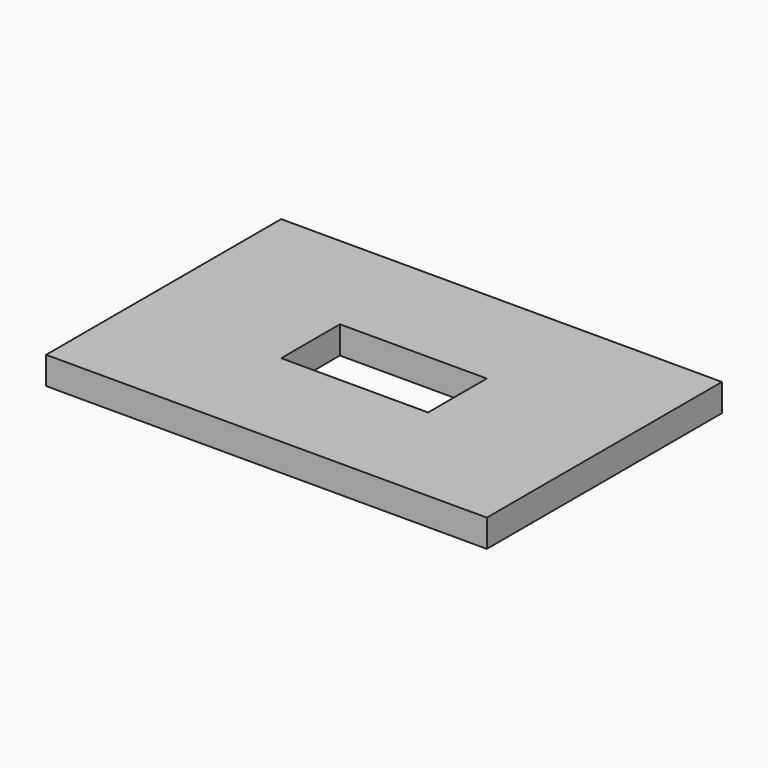
from build123d import *

# Parameters (mm, degrees)
F0_W     = 152.4
F0_H     = 101.6
F0_W_2   = 50.8
F0_H_2   = 25.4
F1_DEPTH = 9.525


# Not quite as in the source:
# - a length typed as a fraction of an inch, garbled in the dataset ("3 / 203.2 mm" for 3/8 in), is restored


with BuildPart() as f1:
    # F0 (on Top) → F1 (new body)
    with BuildSketch(Plane.XY):
        Rectangle(F0_W, F0_H)
        Rectangle(F0_W_2, F0_H_2, mode=Mode.SUBTRACT)
    extrude(amount=F1_DEPTH)


solid = f1.part
